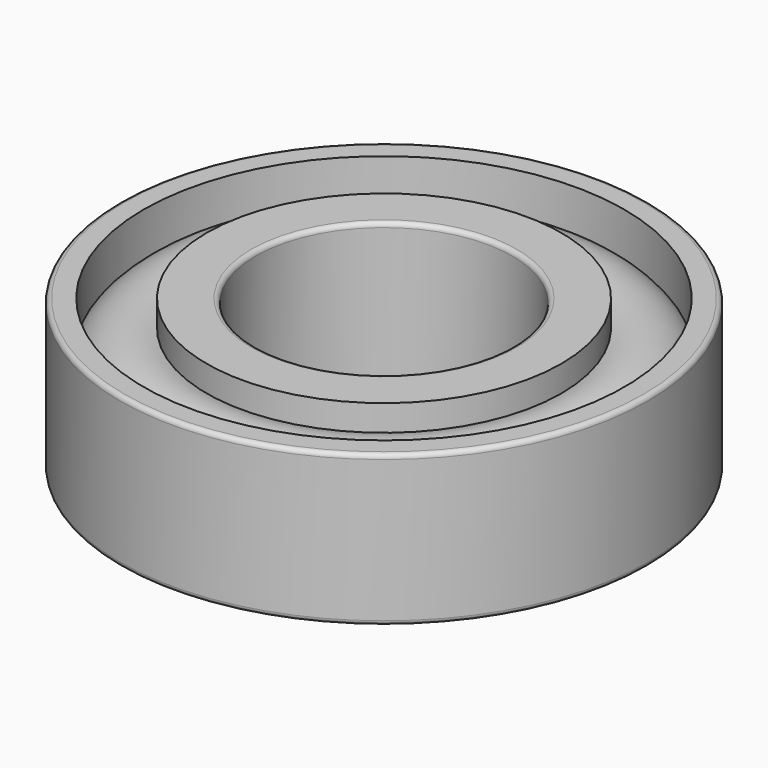
from build123d import *

# Parameters (mm, degrees)
F4_R = 0.3
F5_R = 0.3


with BuildPart() as f3:
    # F2 (on Front) → F3 (revolve)
    with BuildSketch(Plane.XZ):
        with BuildLine():
            Line((-11.75, -5), (-8.5, -5))
            Line((-8.5, -5), (-8.5, 5))
            Line((-8.5, 5), (-11.75, 5))
            Line((-11.75, 5), (-11.75, 3.2691742077))
            ThreePointArc((-11.75, 3.2691742077), (-14.0747440843, 3.3309045548), (-15.925, 1.9220757009))
            Line((-15.925, 1.9220757009), (-15.925, 5))
            Line((-15.925, 5), (-17.5, 5))
            Line((-17.5, 5), (-17.5, -5))
            Line((-17.5, -5), (-15.925, -5))
            Line((-15.925, -5), (-15.925, -1.9220757009))
            ThreePointArc((-15.925, -1.9220757009), (-14.0747440843, -3.3309045548), (-11.75, -3.2691742077))
            Line((-11.75, -3.2691742077), (-11.75, -5))
        make_face()
    revolve(axis=Axis((0, 0, 0), (0, 0, -1)))

    # F4
    f4_edges = [f3.edges().sort_by_distance(p)[0] for p in [
        (17.5, 0, 5),
        (17.5, 0, -5),
    ]]
    fillet(f4_edges, radius=F4_R)

    # F5
    f5_edges = [f3.edges().sort_by_distance(p)[0] for p in [
        (8.5, 0, 5),
        (8.5, 0, -5),
    ]]
    fillet(f5_edges, radius=F5_R)


solid = f3.part
